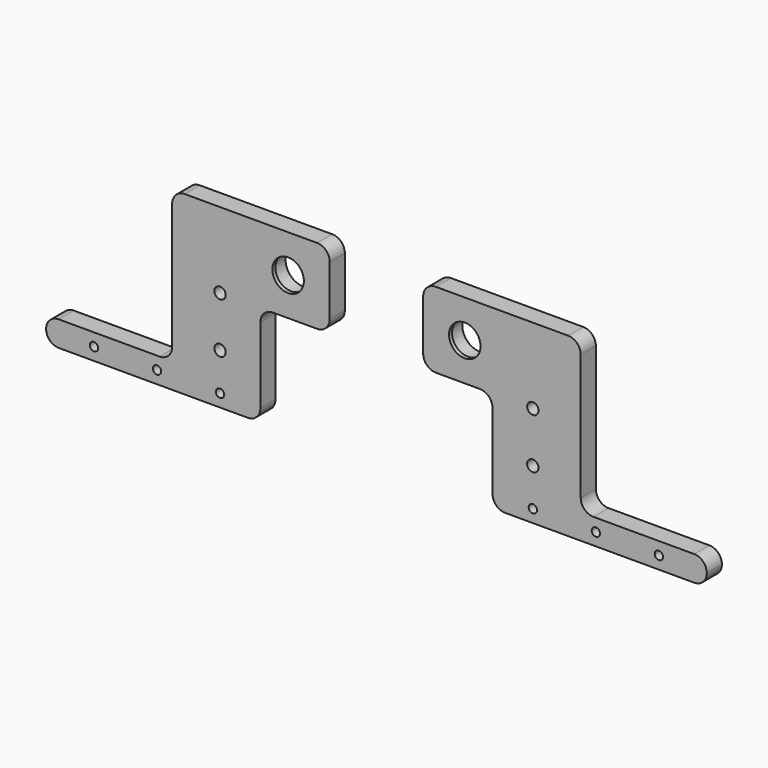
from build123d import *

# Parameters (mm, degrees)
F1_DEPTH       = 15
F2_D           = 9
F3_D           = 6.6
F4_R           = 9.99999
F5_D           = 25
F5_CBORE_D     = 28
F5_CBORE_DEPTH = 12
F6_W           = 40
F6_H           = 80
F7_DEPTH       = 5


# Not quite as in the source:
# - a fillet or chamfer is up to 0.001 mm smaller than in the source, because OpenCascade refuses the exact size


with BuildPart() as f1:
    # F0 (on Front) → F1 (new body)
    with BuildSketch(Plane.XZ):
        Polygon((62.0740194619, 20.9148037434), (-57.9259805381, 20.9148037434), (-62.9259805381, 20.9148037434), (-62.9259805381, -39.0851962566), (-57.9259805381, -39.0851962566), (-7.9259805381, -39.0851962566), (-7.9259805381, -119.0851962566), (162.0740194619, -119.0851962566), (162.0740194619, -99.0851962566), (62.0740194619, -99.0851962566), align=None)
    extrude(amount=F1_DEPTH)

    # F2 (through all)
    with Locations(Plane(origin=(0, 0, 0), x_dir=(1, 0, 0), z_dir=(0, 1, 0))):
        with Locations((24.0740194619, 79.0851962566), (24.0740194619, 39.0851962566)):
            Hole(F2_D / 2)

    # F3 (through all)
    with Locations(Plane(origin=(0, 0, 0), x_dir=(1, 0, 0), z_dir=(0, 1, 0))):
        with Locations((24.0740194619, 109.0851962566), (74.0740194619, 109.0851962566), (124.0740194619, 109.0851962566)):
            Hole(F3_D / 2)

    # F4 (radius 10 in the source; OpenCascade refuses exactly that, so slightly less here)
    f4_edges = [f1.edges().sort_by_distance(p)[0] for p in [
        (62.074019, -7.5, 20.914804),
        (62.074019, -7.5, -99.085196),
        (162.074019, -7.5, -119.085196),
        (162.074019, -7.5, -99.085196),
        (-7.925981, -7.5, -119.085196),
        (-7.925981, -7.5, -39.085196),
        (-62.925981, -7.5, 20.914804),
        (-62.925981, -7.5, -39.085196),
    ]]
    fillet(f4_edges, radius=F4_R)

    # F5 (through all)
    with Locations(Plane(origin=(0, 0, 0), x_dir=(1, 0, 0), z_dir=(0, 1, 0))):
        with Locations((-29.9259805381, 9.0851962566)):
            CounterBoreHole(F5_D / 2, F5_CBORE_D / 2, F5_CBORE_DEPTH)

    # F6 (on face) → F7 (cut)
    with BuildSketch(Plane.XZ):
        with Locations((24.0740194619, -59.0851962566)):
            Rectangle(F6_W, F6_H)
    extrude(amount=F7_DEPTH, mode=Mode.SUBTRACT)


with BuildPart() as f9_1:
    # F9: instance of F1
    add(f1.part.mirror(Plane.YZ.offset(-100)))


solid = Compound([f1.part, f9_1.part])
